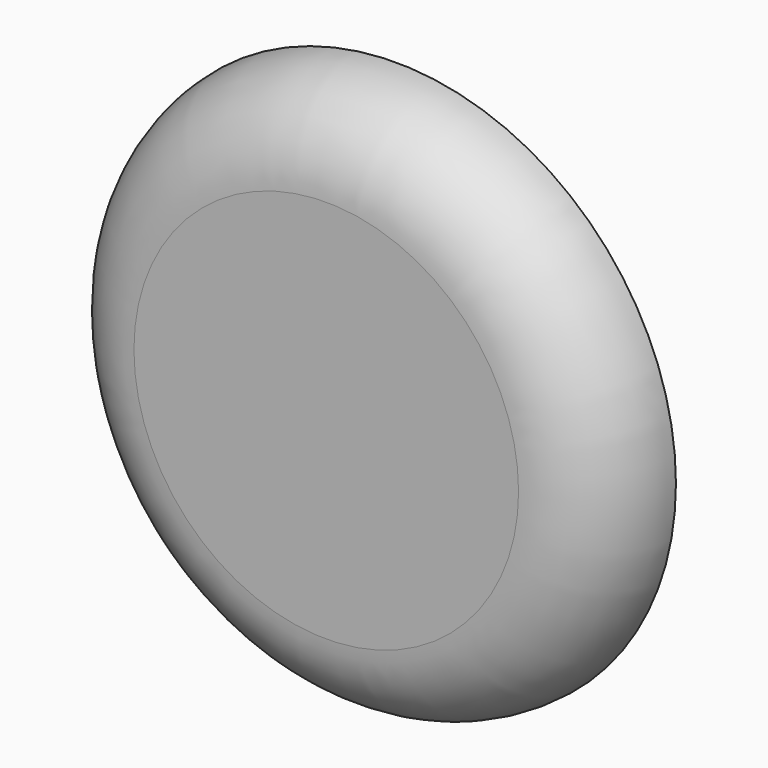
from build123d import *

# Parameters (mm, degrees)
F0_R     = 7.9999967
F1_DEPTH = 2.5
F2_R     = 2.49999
F3_R     = 1.5
F4_DEPTH = 1.25
F5_R     = 2
F6_DEPTH = 1.25
F7_R     = 0.5


# Not quite as in the source:
# - a fillet or chamfer is up to 0.001 mm smaller than in the source, because OpenCascade refuses the exact size


with BuildPart() as f1:
    # F0 (on Front) → F1 (new body)
    with BuildSketch(Plane.XZ):
        Circle(F0_R)
    extrude(amount=F1_DEPTH)

    # F2 (radius 2.5 in the source; OpenCascade refuses exactly that, so slightly less here)
    f2_edges = [f1.edges().sort_by_distance(p)[0] for p in [
        (-7.999997, -2.5, 0),
    ]]
    fillet(f2_edges, radius=F2_R)


with BuildPart() as f4:
    # F3 (on Front) → F4 (new body)
    with BuildSketch(Plane.XZ):
        Circle(F3_R)
    extrude(amount=-F4_DEPTH)

    # F5 (on face) → F6 (join)
    with BuildSketch(Plane(origin=(0, 1.25, 0), x_dir=(-1, 0, 0), z_dir=(0, 1, 0))):
        Circle(F5_R)
    extrude(amount=F6_DEPTH)

    # F7
    f7_edges = [f4.edges().sort_by_distance(p)[0] for p in [
        (2, 2.5, 0),
    ]]
    fillet(f7_edges, radius=F7_R)


solid = Compound([f1.part, f4.part])
